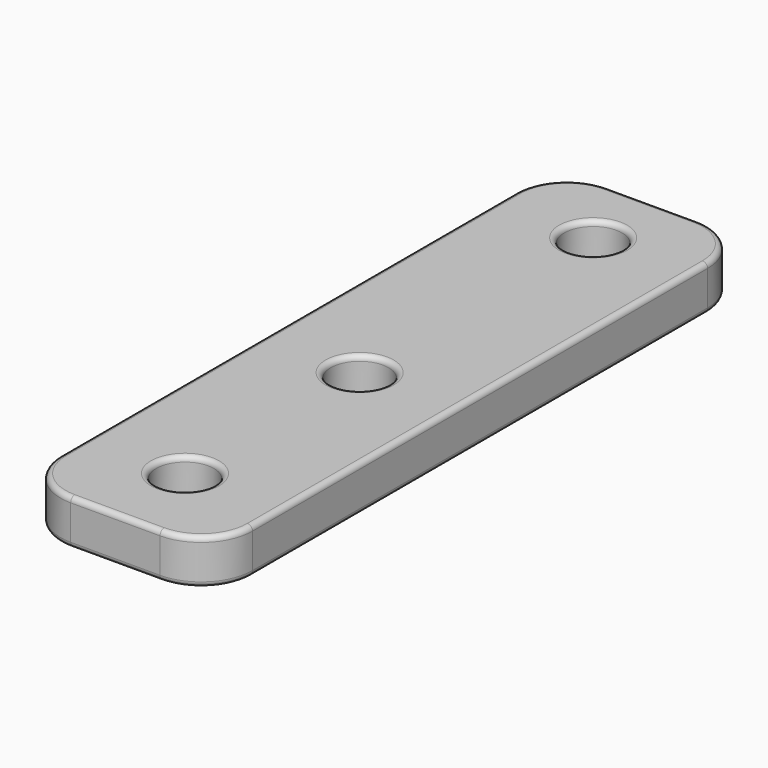
from build123d import *

# Parameters (mm, degrees)
F0_R     = 2.8575
F0_W     = 19
F0_H     = 20.7006
F1_DEPTH = 4.445
F2_R     = 5.08
F3_R     = 0.508


# Not quite as in the source:
# - a feature names something its author has since deleted; it is built from what else it names


with BuildPart() as f1:
    # F0 (on Top) → F1 (new body)
    with BuildSketch(Plane.XY):
        Polygon((-19, 0), (0, 0), (0, 45.72), (-19, 45.72), (-19, 19), align=None)
        with Locations((-9.5, 9.5)):
            Circle(F0_R, mode=Mode.SUBTRACT)
        with Locations((-9.5, 38.3675)):
            Circle(F0_R, mode=Mode.SUBTRACT)
        with Locations((-9.5, -10.3503)):
            Rectangle(F0_W, F0_H)
        with Locations((-9.5, -12.09)):
            Circle(F0_R, mode=Mode.SUBTRACT)
    extrude(amount=F1_DEPTH)

    # F2
    f2_edges = [f1.edges().sort_by_distance(p)[0] for p in [
        (0, 45.72, 2.2225),
        (-19, 45.72, 2.2225),
        (0, -20.7006, 2.2225),
        (-19, -20.7006, 2.2225),
    ]]
    fillet(f2_edges, radius=F2_R)

    # F3
    f3_edges = [f1.edges().sort_by_distance(p)[0] for p in [
        (0, 12.5097, 4.445),
        (-12.3575, 9.5, 4.445),
        (-12.3575, 38.3675, 4.445),
        (0, 12.5097, 0),
        (-12.3575, 9.5, 0),
        (-12.3575, -12.09, 4.445),
        (-12.3575, -12.09, 0),
        (-12.3575, 38.3675, 0),
        (-9.5, 45.72, 0),
        (-9.5, 45.72, 4.445),
        (-1.487898, 44.232102, 0),
        (-17.512102, 44.232102, 0),
        (-19, 12.5097, 0),
        (-1.487898, -19.212702, 0),
        (-17.512102, -19.212702, 0),
        (-9.5, -20.7006, 0),
        (-1.487898, 44.232102, 4.445),
        (-17.512102, 44.232102, 4.445),
        (-19, 12.5097, 4.445),
        (-1.487898, -19.212702, 4.445),
        (-17.512102, -19.212702, 4.445),
        (-9.5, -20.7006, 4.445),
    ]]
    fillet(f3_edges, radius=F3_R)


solid = f1.part
